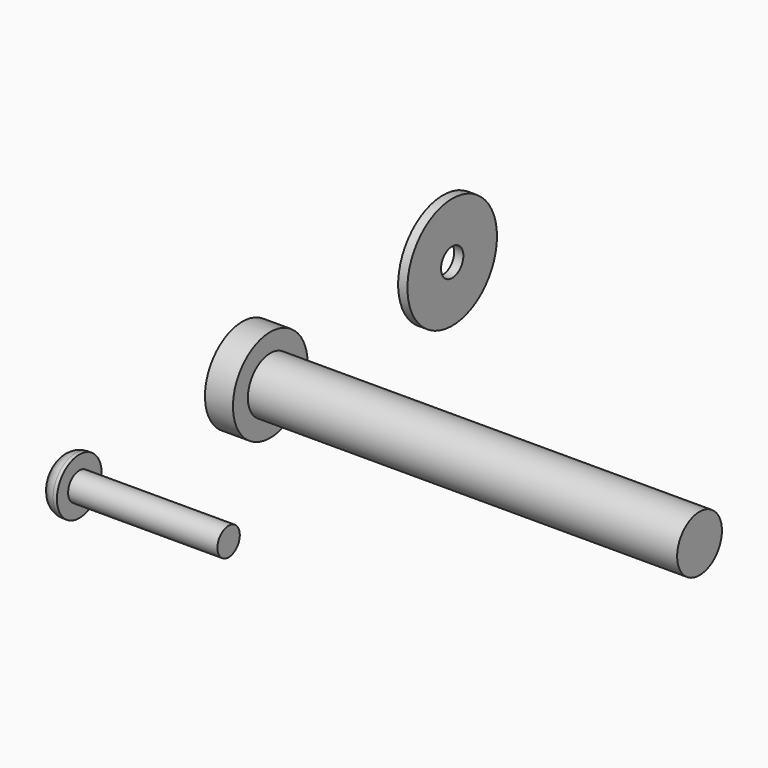
from build123d import *

# Parameters (mm, degrees)
F0_R      = 7.9375
F1_DEPTH  = 4.7625
F2_R      = 4.7625
F3_DEPTH  = 73.025
F4_R      = 2.38125
F5_DEPTH  = 25.4
F6_R      = 9.525
F6_R_2    = 2.3749
F7_DEPTH  = 1.5748
F8_R      = 4.7625
F9_DEPTH  = 3.175
F10_R     = 2.38125
F11_DEPTH = 25.4


# Not quite as in the source:
# - a fillet or chamfer that OpenCascade refuses, or shapes differently, is made with other operations: its cross-section is extruded or revolved along the edge and cut away or added


with BuildPart() as f1:
    # F0 (on Right) → F1 (new body)
    with BuildSketch(Plane.YZ):
        Circle(F0_R)
    extrude(amount=F1_DEPTH)

    # F2 (on face) → F3 (join)
    with BuildSketch(Plane.YZ.offset(4.7625)):
        Circle(F2_R)
    extrude(amount=F3_DEPTH)

    # F4 (on face) → F5 (cut)
    with BuildSketch(Plane(origin=(0, 0, 0), x_dir=(0, -1, 0), z_dir=(-1, 0, 0))):
        Circle(F4_R)
    extrude(amount=-F5_DEPTH, mode=Mode.SUBTRACT)


with BuildPart() as f7:
    # F6 (on Right) → F7 (new body)
    with BuildSketch(Plane.YZ):
        with Locations((42.671024815, 0)):
            Circle(F6_R)
        with Locations((42.671024815, 0)):
            Circle(F6_R_2, mode=Mode.SUBTRACT)
    extrude(amount=F7_DEPTH)


with BuildPart() as f9:
    # F8 (on Right) → F9 (new body)
    with BuildSketch(Plane.YZ):
        with Locations((-38.6279119517, 0)):
            Circle(F8_R)
        Polygon((-36.9000906235, -1.5874504059), (-39.1387736664, -2.2900623664), (-40.8665949945, -0.7026119604), (-40.3557332798, 1.5874504059), (-38.117050237, 2.2900623664), (-36.3892289088, 0.7026119604), align=None, mode=Mode.SUBTRACT)
    extrude(amount=F9_DEPTH)

    # F10 (on face) → F11 (join)
    with BuildSketch(Plane.YZ.offset(3.175)):
        with Locations((-38.6279119517, 0)):
            Circle(F10_R)
        Polygon((-40.3557332798, 1.5874504059), (-38.117050237, 2.2900623664), (-36.3892289088, 0.7026119604), (-36.9000906235, -1.5874504059), (-39.1387736664, -2.2900623664), (-40.8665949945, -0.7026119604), align=None, mode=Mode.SUBTRACT)
        Polygon((-36.3892289088, 0.7026119604), (-38.117050237, 2.2900623664), (-40.3557332798, 1.5874504059), (-40.8665949945, -0.7026119604), (-39.1387736664, -2.2900623664), (-36.9000906235, -1.5874504059), align=None)
    extrude(amount=F11_DEPTH)

    # F12: fillet of radius 2.54 on 1 edges, made by hand

    # F12_s1 → F12_t2 (revolve, cut)
    with BuildSketch(Plane.XY):
        with BuildLine():
            ThreePointArc((2.54, -33.8654119517), (0.7439487758, -34.6093607275), (0, -36.4054119517))
            Line((0, -36.4054119517), (0, -33.8654119517))
            Line((0, -33.8654119517), (2.54, -33.8654119517))
        make_face()
    revolve(axis=Axis((0, -38.6279119517, 0), (1, 0, 0)), mode=Mode.SUBTRACT)


solid = Compound([f1.part, f7.part, f9.part])
